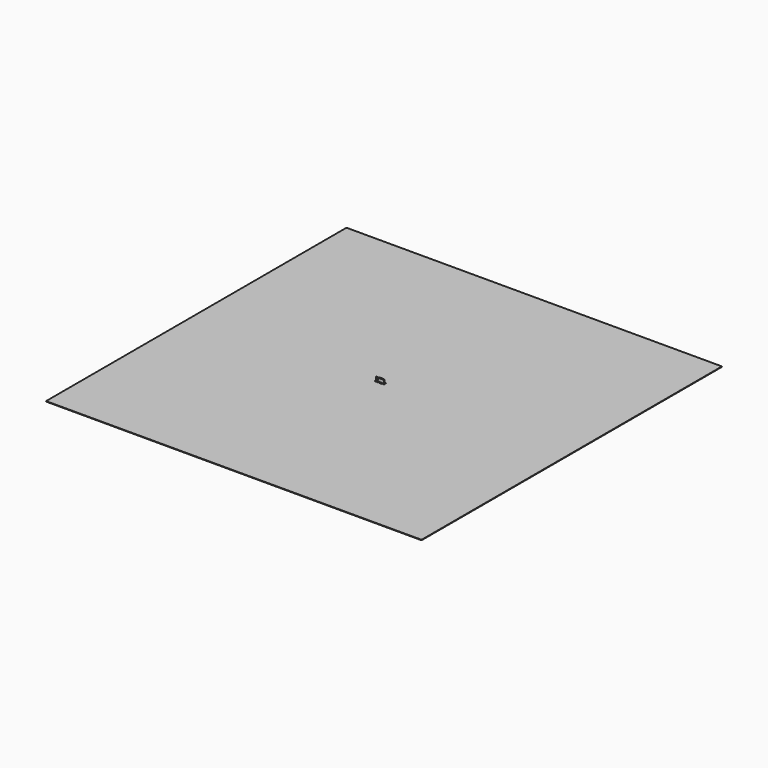
from build123d import *

# Parameters (mm, degrees)
F1_DEPTH = 838.2
F3_DEPTH = 152.4
F4_W     = 6221.8872991562
F4_H     = 1921.1952090263
F4_W_2   = 6018.6872991562
F4_H_2   = 1717.9952090263
F5_DEPTH = 127
F6_W     = 254000
F6_H     = 254000
F6_W_2   = 5486.4
F6_H_2   = 304.8
F7_DEPTH = 304.8


# Not quite as in the source:
# - a feature names something its author has since deleted; it is built from what else it names


with BuildPart() as f1:
    # F0 (on Top) → F1 (new body, symmetric)
    with BuildSketch(Plane.XY):
        with BuildLine():
            Line((-152.4, 152.4), (-152.4, 0))
            Line((-152.4, 0), (-152.4, -152.4))
            ThreePointArc((-152.4, -152.4), (1943.1, -457.2), (4038.6, -152.4))
            Line((4038.6, -152.4), (4038.6, 152.4))
            ThreePointArc((4038.6, 152.4), (1943.1, 457.2), (-152.4, 152.4))
        make_face()
    extrude(amount=F1_DEPTH, both=True)


with BuildPart() as f3:
    # F2 (on Front) → F3 (new body, symmetric)
    with BuildSketch(Plane.XZ):
        Polygon((-228.6, -939.8), (-228.6, 0), (-228.6, 838.2), (-1447.8, 838.2), (-1447.8, -1549.4), (4038.6, -1549.4), (4038.6, -939.8), align=None)
    extrude(amount=F3_DEPTH, both=True)


with BuildPart() as f5:
    # F4 (on face) → F5 (new body, symmetric)
    with BuildSketch(Plane(origin=(0, 0, -1549.4), x_dir=(1, 0, 0), z_dir=(0, 0, -1))):
        with Locations((1444.4946988106, 9.7524821758)):
            Rectangle(F4_W, F4_H)
        with Locations((1444.4946988106, 9.7524821758)):
            Rectangle(F4_W_2, F4_H_2, mode=Mode.SUBTRACT)
    extrude(amount=F5_DEPTH, both=True)


with BuildPart() as f7:
    # F6 (on face) → F7 (new body)
    with BuildSketch(Plane(origin=(0, 0, -1549.4), x_dir=(1, 0, 0), z_dir=(0, 0, -1))):
        with Locations((4038.6, 152.4)):
            Rectangle(F6_W, F6_H)
        with Locations((1295.4, 0)):
            Rectangle(F6_W_2, F6_H_2, mode=Mode.SUBTRACT)
    extrude(amount=F7_DEPTH)


solid = Compound([f1.part, f3.part, f5.part, f7.part])
